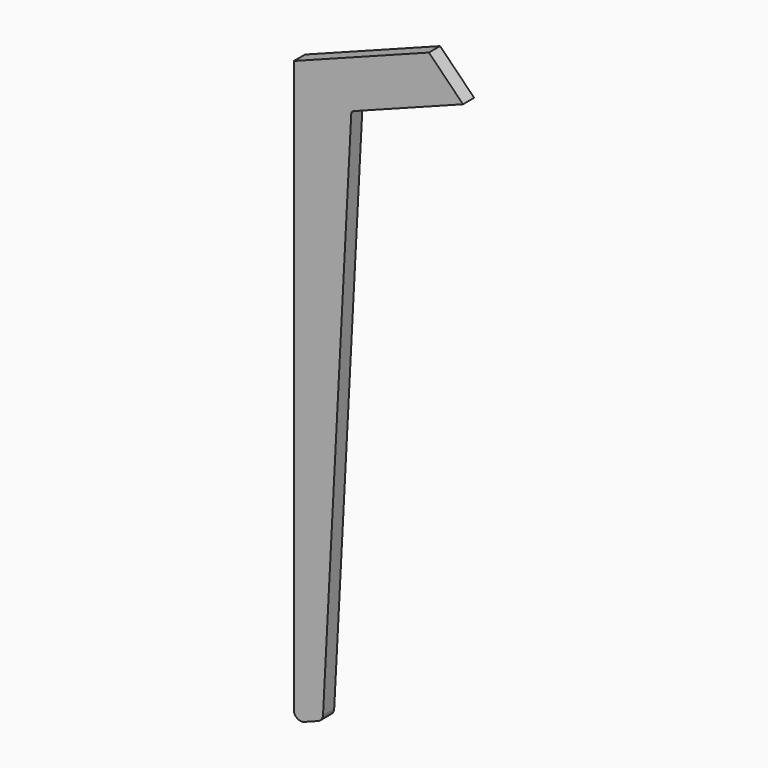
from build123d import *

# Parameters (mm, degrees)
F0_R     = 3
F1_DEPTH = 18
F2_DEPTH = 14
F3_DEPTH = 12.5


# Not quite as in the source:
# - ends of sketch curves that miss each other by under 0.0002 mm in the source are joined


with BuildPart() as f1:
    # F0 (on Front) → F1 (new body)
    with BuildSketch(Plane.XZ):
        with BuildLine():
            Line((-119.3285324557, -448.2617723394), (-101.6685144557, -441.5452453394))
            ThreePointArc((-101.6685144557, -441.5452453394), (-97.1422559669, -438.0887567531), (-95.2370421293, -432.7217753041))
            Line((-95.2370421293, -432.7217753041), (-58.8235234557, 262.0895416606))
            ThreePointArc((-58.8235234557, 262.0895416606), (-58.06143799, 264.2363343101), (-56.250934498, 265.6189297718))
            Line((-56.250934498, 265.6189297718), (85.2578445443, 319.4380986606))
            Line((85.2578445443, 319.4380986606), (41.3370915443, 363.9049416606))
            Line((41.3370915443, 363.9049416606), (-132.8833544557, 297.6447436606))
            Line((-132.8833544557, 297.6447436606), (-132.8833544557, -438.9149423394))
            ThreePointArc((-132.8833544557, -438.9149423394), (-128.5601395631, -447.1474456551), (-119.3285324557, -448.2617723394))
        make_face()
        with Locations((-116.1363294557, -390.4994083394)):
            Circle(F0_R, mode=Mode.SUBTRACT)
        with Locations((-113.3511164557, -246.7075803394)):
            Circle(F0_R, mode=Mode.SUBTRACT)
        with Locations((-107.9187374557, -78.3756793394)):
            Circle(F0_R, mode=Mode.SUBTRACT)
        with Locations((-105.9467734557, 128.6347116606)):
            Circle(F0_R, mode=Mode.SUBTRACT)
        with Locations((-99.7011464557, 233.7480486606)):
            Circle(F0_R, mode=Mode.SUBTRACT)
        with Locations((-120.2235504557, 275.4892296606)):
            Circle(F0_R, mode=Mode.SUBTRACT)
        with BuildLine():
            ThreePointArc((-90.3754553764, 255.7239337355), (-90.5472879726, 250.0640248228), (-96.2068413545, 250.2471937553))
            Line((-96.2068413545, 250.2471937553), (-102.4861304557, 250.4567146606))
            ThreePointArc((-102.4861304557, 250.4567146606), (-108.1617141765, 250.6689360163), (-107.9038666822, 256.3426299107))
            Line((-107.9038666822, 256.3426299107), (-107.0299454557, 291.0352376606))
            ThreePointArc((-107.0299454557, 291.0352376606), (-106.7545815371, 296.6558621202), (-101.1313975225, 296.4389595982))
            Line((-101.1313975225, 296.4389595982), (-94.4508164557, 296.2088706606))
            ThreePointArc((-94.4508164557, 296.2088706606), (-88.7851572097, 296.0073908544), (-89.0114747479, 290.3426689785))
            Line((-89.0114747479, 290.3426689785), (-90.3754553764, 255.7239337355))
        make_face(mode=Mode.SUBTRACT)
        with Locations((-42.3545774557, 288.6199666606)):
            Circle(F0_R, mode=Mode.SUBTRACT)
        with Locations((51.7271015443, 324.4037386606)):
            Circle(F0_R, mode=Mode.SUBTRACT)
        with Locations((-116.1363294557, -390.4994083394)):
            Circle(F0_R)
        with Locations((-113.3511164557, -246.7075803394)):
            Circle(F0_R)
        with Locations((-107.9187374557, -78.3756793394)):
            Circle(F0_R)
        with Locations((-105.9467734557, 128.6347116606)):
            Circle(F0_R)
        with Locations((-120.2235504557, 275.4892296606)):
            Circle(F0_R)
        with Locations((-99.7011464557, 233.7480486606)):
            Circle(F0_R)
        with Locations((-42.3545774557, 288.6199666606)):
            Circle(F0_R)
        with Locations((51.7271015443, 324.4037386606)):
            Circle(F0_R)
        with BuildLine():
            Line((-102.4861304557, 250.4567146606), (-96.2068414557, 250.2471936606))
            ThreePointArc((-96.2068414557, 250.2471936606), (-90.5472879726, 250.0640248228), (-90.3754553764, 255.7239337355))
            Line((-90.3754553764, 255.7239337355), (-89.0114744557, 290.3426686606))
            ThreePointArc((-89.0114744557, 290.3426686606), (-88.7851572097, 296.0073908544), (-94.4508168599, 296.2088710928))
            Line((-94.4508168599, 296.2088710928), (-101.1313974557, 296.4389596606))
            ThreePointArc((-101.1313974557, 296.4389596606), (-106.7545815371, 296.6558621202), (-107.0299455087, 291.0352376131))
            Line((-107.0299455087, 291.0352376131), (-107.9038664557, 256.3426296606))
            ThreePointArc((-107.9038664557, 256.3426296606), (-108.1617141765, 250.6689360163), (-102.4861304557, 250.4567146606))
        make_face()
    extrude(amount=F1_DEPTH)

    # F0 (on Front) → F2 (cut)
    with BuildSketch(Plane.XZ):
        with Locations((-116.1363294557, -390.4994083394)):
            Circle(F0_R)
        with Locations((-113.3511164557, -246.7075803394)):
            Circle(F0_R)
        with Locations((-107.9187374557, -78.3756793394)):
            Circle(F0_R)
        with Locations((-105.9467734557, 128.6347116606)):
            Circle(F0_R)
        with Locations((-120.2235504557, 275.4892296606)):
            Circle(F0_R)
        with Locations((-99.7011464557, 233.7480486606)):
            Circle(F0_R)
        with Locations((-42.3545774557, 288.6199666606)):
            Circle(F0_R)
        with Locations((51.7271015443, 324.4037386606)):
            Circle(F0_R)
    extrude(amount=F2_DEPTH, mode=Mode.SUBTRACT)

    # F0 (on Front) → F3 (cut)
    with BuildSketch(Plane.XZ):
        with BuildLine():
            Line((-102.4861304557, 250.4567146606), (-96.2068414557, 250.2471936606))
            ThreePointArc((-96.2068414557, 250.2471936606), (-90.5472879726, 250.0640248228), (-90.3754553764, 255.7239337355))
            Line((-90.3754553764, 255.7239337355), (-89.0114744557, 290.3426686606))
            ThreePointArc((-89.0114744557, 290.3426686606), (-88.7851572097, 296.0073908544), (-94.4508168599, 296.2088710928))
            Line((-94.4508168599, 296.2088710928), (-101.1313974557, 296.4389596606))
            ThreePointArc((-101.1313974557, 296.4389596606), (-106.7545815371, 296.6558621202), (-107.0299455087, 291.0352376131))
            Line((-107.0299455087, 291.0352376131), (-107.9038664557, 256.3426296606))
            ThreePointArc((-107.9038664557, 256.3426296606), (-108.1617141765, 250.6689360163), (-102.4861304557, 250.4567146606))
        make_face()
    extrude(amount=F3_DEPTH, mode=Mode.SUBTRACT)


solid = f1.part
